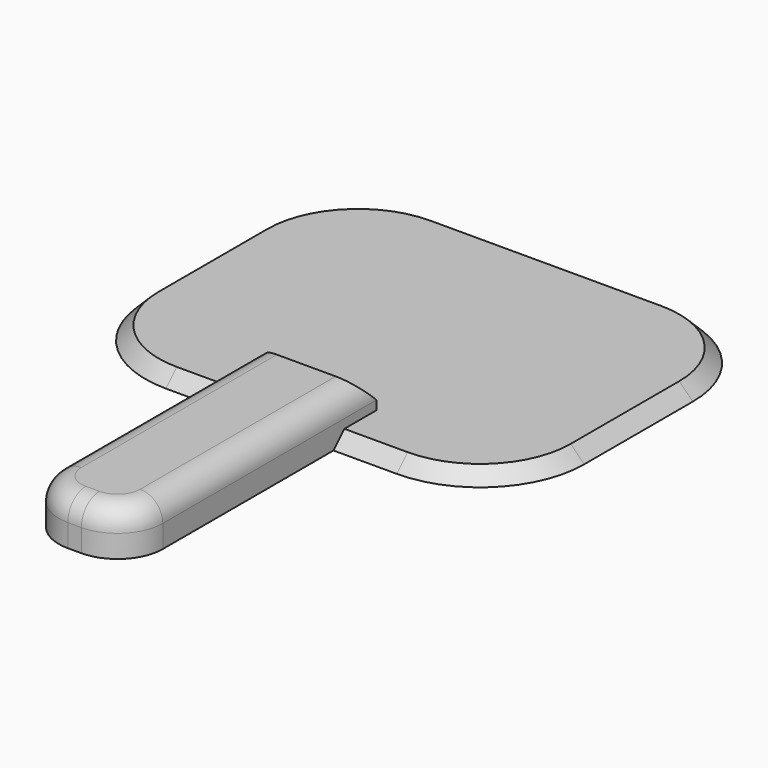
from build123d import *

# Parameters (mm, degrees)
F0_W         = 101
F0_H         = 80
F1_DEPTH     = 3
F2_R         = 25
F3_W         = 23
F3_H         = 69
F4_DEPTH     = 10
F5_R         = 10
F6_SIZE      = 5
F7_R         = 5
F8_T1_DEPTH  = 30
F8_T3_DEPTH  = 51
F8_T5_DEPTH  = 14
F8_T7_DEPTH  = 14
F8_T10_ANGLE = 90
F8_T12_ANGLE = 90
F8_T14_ANGLE = 90
F8_T16_ANGLE = 90


# Not quite as in the source:
# - a fillet or chamfer that OpenCascade refuses, or shapes differently, is made with other operations: its cross-section is extruded or revolved along the edge and cut away or added


with BuildPart() as f1:
    # F0 (on Top) → F1 (new body)
    with BuildSketch(Plane.XY):
        with Locations((0, 33.399283886)):
            Rectangle(F0_W, F0_H)
    extrude(amount=F1_DEPTH)

    # F2
    f2_edges = [f1.edges().sort_by_distance(p)[0] for p in [
        (50.5, -6.600716, 1.5),
        (50.5, 73.399284, 1.5),
        (-50.5, -6.600716, 1.5),
        (-50.5, 73.399284, 1.5),
    ]]
    fillet(f2_edges, radius=F2_R)

    # F3 (on Top) → F4 (join)
    with BuildSketch(Plane.XY):
        with Locations((0, -27.2368434817)):
            Rectangle(F3_W, F3_H)
    extrude(amount=F4_DEPTH)

    # F5
    f5_edges = [f1.edges().sort_by_distance(p)[0] for p in [
        (11.5, -61.736843, 5),
        (-11.5, -61.736843, 5),
    ]]
    fillet(f5_edges, radius=F5_R)

    # F6
    f6_edges = [f1.edges().sort_by_distance(p)[0] for p in [
        (0, 7.263157, 10),
    ]]
    chamfer(f6_edges, length=F6_SIZE)

    # F7
    f7_edges = [f1.edges().sort_by_distance(p)[0] for p in [
        (-11.5, -24.736843, 10),
    ]]
    fillet(f7_edges, radius=F7_R)

    # F8: chamfer of 5 on 1 edges, made by hand

    # F8_s2 → F8_t1 (cut)
    with BuildSketch(Plane.XZ.offset(-48.399283886)):
        Polygon((-45.5, 3), (-50.5, -2), (-50.5, 3), align=None)
        Polygon((45.5, 3), (50.5, -2), (50.5, 3), align=None)
    extrude(amount=F8_T1_DEPTH, mode=Mode.SUBTRACT)

    # F8_s4 → F8_t3 (cut)
    with BuildSketch(Plane.YZ.offset(-25.5)):
        Polygon((68.399283886, 3), (73.399283886, -2), (73.399283886, 3), align=None)
    extrude(amount=F8_T3_DEPTH, mode=Mode.SUBTRACT)

    # F8_s6 → F8_t5 (cut)
    with BuildSketch(Plane.YZ.offset(11.5)):
        Polygon((-1.600716114, 3), (-6.600716114, -2), (-6.600716114, 3), align=None)
    extrude(amount=F8_T5_DEPTH, mode=Mode.SUBTRACT)

    # F8_s8 → F8_t7 (cut)
    with BuildSketch(Plane.YZ.offset(-25.5)):
        Polygon((-6.600716114, -2), (-1.600716114, 3), (-6.600716114, 3), align=None)
    extrude(amount=F8_T7_DEPTH, mode=Mode.SUBTRACT)

    # F8_s9 → F8_t10 (revolve, cut)
    with BuildSketch(Plane.XZ.offset(-48.399283886)):
        Polygon((-45.5, 3), (-50.5, -2), (-50.5, 3), align=None)
    revolve(axis=Axis((-25.5, 48.399283886, 3), (0, 0, -1)), revolution_arc=F8_T10_ANGLE, mode=Mode.SUBTRACT)

    # F8_s11 → F8_t12 (revolve, cut)
    with BuildSketch(Plane.XZ.offset(-48.399283886)):
        Polygon((45.5, 3), (50.5, -2), (50.5, 3), align=None)
    revolve(axis=Axis((25.5, 48.399283886, 3), (0, 0, 1)), revolution_arc=F8_T12_ANGLE, mode=Mode.SUBTRACT)

    # F8_s13 → F8_t14 (revolve, cut)
    with BuildSketch(Plane.YZ.offset(25.5)):
        Polygon((-1.600716114, 3), (-6.600716114, -2), (-6.600716114, 3), align=None)
    revolve(axis=Axis((25.5, 18.399283886, 3), (0, 0, 1)), revolution_arc=F8_T14_ANGLE, mode=Mode.SUBTRACT)

    # F8_s15 → F8_t16 (revolve, cut)
    with BuildSketch(Plane.XZ.offset(-18.399283886)):
        Polygon((-45.5, 3), (-50.5, -2), (-50.5, 3), align=None)
    revolve(axis=Axis((-25.5, 18.399283886, 3), (0, 0, 1)), revolution_arc=F8_T16_ANGLE, mode=Mode.SUBTRACT)


solid = f1.part
